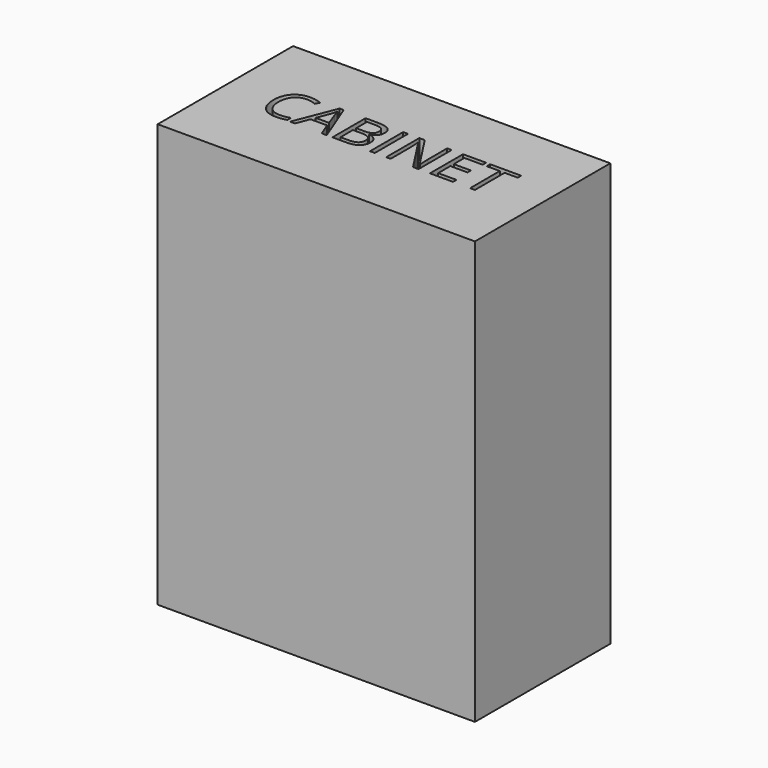
from build123d import *

# Parameters (mm, degrees)
F0_W         = 1500
F0_H         = 800
F1_DEPTH     = 2000
F2_TEXT_SIZE = 274.2268041604
F3_DEPTH     = 92


# Not quite as in the source:
# - Text() gives the source's letters only with a copy of the font that has no kerning and outlines rounded to 1/6400 em; it was checked with that copy


with BuildPart() as f1:
    # F0 (on Top) → F1 (new body)
    with BuildSketch(Plane.XY):
        Rectangle(F0_W, F0_H)
    extrude(amount=F1_DEPTH)

    # F2 (on face) → F3 (cut)
    with BuildSketch(Plane.XY.offset(2000)):
        with Locations((-554.2268157005, -78.804127872)):
            Text('CABINET', F2_TEXT_SIZE, font='Open Sans', text_align=(TextAlign.LEFT, TextAlign.BOTTOM))
    extrude(amount=-F3_DEPTH, mode=Mode.SUBTRACT)


solid = f1.part
